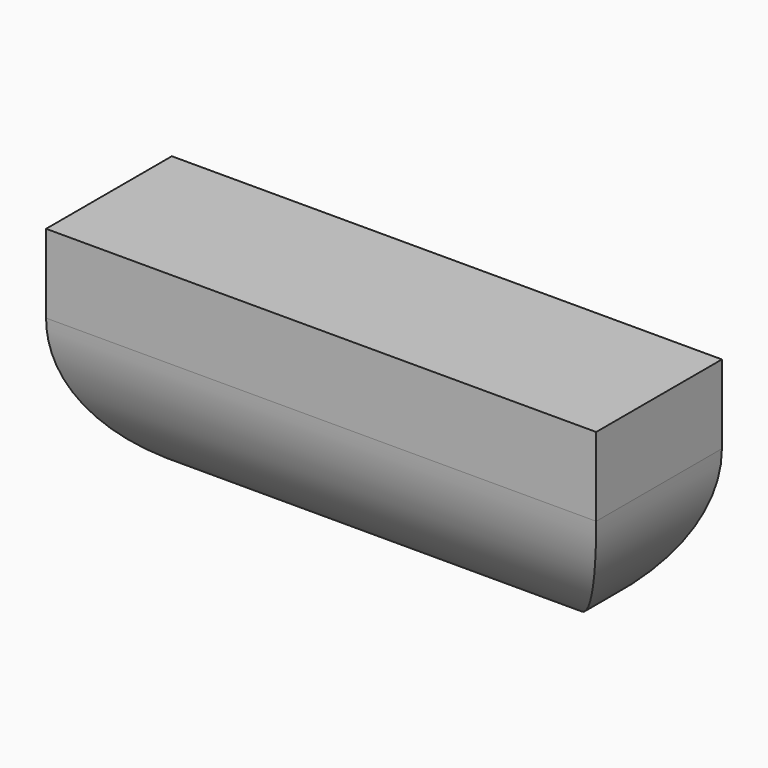
from build123d import *

# Parameters (mm, degrees)
F0_W        = 88.9
F0_H        = 38.1
F1_DEPTH    = 25.4
F2_T1_DEPTH = 152.4
F2_T3_DEPTH = 215.9


# Not quite as in the source:
# - a fillet or chamfer that OpenCascade refuses, or shapes differently, is made with other operations: its cross-section is extruded or revolved along the edge and cut away or added


with BuildPart() as f1:
    # F0 (on Front) → F1 (new body)
    with BuildSketch(Plane.XZ):
        Rectangle(F0_W, F0_H)
    extrude(amount=F1_DEPTH)

    # F2: fillet of radius 25.4 on 4 edges, made by hand

    # F2_s2 → F2_t1 (cut)
    with BuildSketch(Plane.XZ.offset(-63.5)):
        with BuildLine():
            ThreePointArc((44.45, 6.35), (37.0105122421, -11.6105122421), (19.05, -19.05))
            Line((19.05, -19.05), (44.45, -19.05))
            Line((44.45, -19.05), (44.45, 6.35))
        make_face()
        with BuildLine():
            ThreePointArc((-44.45, 6.35), (-37.0105122421, -11.6105122421), (-19.05, -19.05))
            Line((-19.05, -19.05), (-44.45, -19.05))
            Line((-44.45, -19.05), (-44.45, 6.35))
        make_face()
    extrude(amount=F2_T1_DEPTH, mode=Mode.SUBTRACT)

    # F2_s4 → F2_t3 (cut)
    with BuildSketch(Plane.YZ.offset(-107.95)):
        with BuildLine():
            ThreePointArc((0, -19.05), (-17.9605122421, -11.6105122421), (-25.4, 6.35))
            Line((-25.4, 6.35), (-25.4, -19.05))
            Line((-25.4, -19.05), (0, -19.05))
        make_face()
        with BuildLine():
            ThreePointArc((-25.4, -19.05), (-7.4394877579, -11.6105122421), (0, 6.35))
            Line((0, 6.35), (0, -19.05))
            Line((0, -19.05), (-25.4, -19.05))
        make_face()
    extrude(amount=F2_T3_DEPTH, mode=Mode.SUBTRACT)


solid = f1.part
